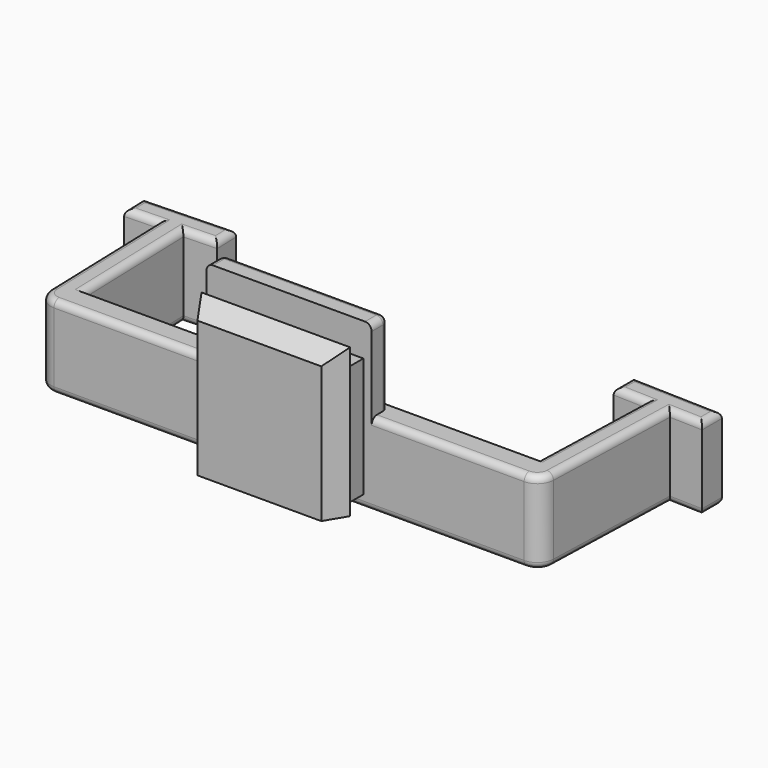
from build123d import *

# Parameters (mm, degrees)
F1_DEPTH      = 10
F3_DEPTH      = 10
F4_DEPTH      = 9
F5_DEPTH      = 9
F6_SIZE2      = 2.49999
F6_SIZE       = 1.49999
F7_R          = 0.8
F8_R          = 0.8
F9_R          = 0.8
F10_T1_DEPTH  = 10
F10_T4_ANGLE  = 88.2100893918
F10_T6_ANGLE  = 88.2100893918
F10_T8_ANGLE  = 88.2100893918
F10_T10_ANGLE = 88.2100893918


# Not quite as in the source:
# - a fillet or chamfer that OpenCascade refuses, or shapes differently, is made with other operations: its cross-section is extruded or revolved along the edge and cut away or added
# - a fillet or chamfer is up to 0.001 mm smaller than in the source, because OpenCascade refuses the exact size


with BuildPart() as f1:
    # F0 (on Top) → F1 (new body)
    with BuildSketch(Plane.XY):
        Polygon((27.5, 0), (-27.5, 0), (-28, 16), (-30.9985362283, 15.9062957429), (-30.4077144863, -3), (30.4077144863, -3), (30.9985362283, 15.9062957429), (28, 16), align=None)
        Polygon((-30.9985362283, 15.9062957429), (-28, 16), (-24.0019516957, 16.1249390095), (-24.0956559528, 19.1234752378), (-35.0902887897, 18.7798929616), (-34.9965845326, 15.7813567334), align=None)
        Polygon((24.0019516957, 16.1249390095), (28, 16), (30.9985362283, 15.9062957429), (34.9965845326, 15.7813567334), (34.9965845326, 18.7813567334), (24.0019516957, 19.1249390095), align=None)
    extrude(amount=F1_DEPTH)

    # F2 (on Right) → F3 (join, symmetric)
    with BuildSketch(Plane.YZ):
        Polygon((-3, 16), (-3, 10), (-0.5, 10), (-0.5, 20), (-3, 20), align=None)
    extrude(amount=F3_DEPTH, both=True)

    # F2 (on Right) → F4 (join, symmetric)
    with BuildSketch(Plane.YZ):
        Polygon((-3, 1.5), (-3, 10), (-3, 16), (-5, 16), (-5, 1.5), align=None)
    extrude(amount=F4_DEPTH, both=True)

    # F2 (on Right) → F5 (join, symmetric)
    with BuildSketch(Plane.YZ):
        Polygon((-5, 0), (-5, 1.5), (-5, 16), (-5, 18), (-7.5, 18), (-7.5, 0), align=None)
    extrude(amount=F5_DEPTH, both=True)

    # F6 (size 1.5 and 2.5 in the source; OpenCascade refuses exactly that, so slightly less here)
    f6_edges = [f1.edges().sort_by_distance(p)[0] for p in [
        (0, -7.5, 18),
        (-9, -7.5, 9),
        (9, -7.5, 9),
    ]]
    f6_side = f1.faces().sort_by_distance((0, -7.5, 9))[0]
    chamfer(f6_edges, length=F6_SIZE, length2=F6_SIZE2, reference=f6_side)

    # F7
    f7_edges = [f1.edges().sort_by_distance(p)[0] for p in [
        (27.75, 8, 0),
        (0, 0, 0),
        (-27.75, 8, 0),
        (-26.000976, 16.06247, 0),
        (-24.048804, 17.624207, 0),
        (-29.592972, 18.951684, 0),
        (-35.043437, 17.280625, 0),
        (-32.99756, 15.843826, 0),
        (-30.703125, 6.453148, 0),
        (0, -3, 0),
        (30.703125, 6.453148, 0),
        (32.99756, 15.843826, 0),
        (34.996585, 17.281357, 0),
        (29.499268, 18.953148, 0),
        (24.001952, 17.624939, 0),
        (26.000976, 16.06247, 0),
    ]]
    fillet(f7_edges, radius=F7_R)

    # F8
    f8_edges = [f1.edges().sort_by_distance(p)[0] for p in [
        (-29.592972, 18.951684, 10),
        (-35.043437, 17.280625, 10),
        (-32.99756, 15.843826, 10),
        (-26.000976, 16.06247, 10),
        (-24.048804, 17.624207, 10),
        (-27.75, 8, 10),
        (-30.703125, 6.453148, 10),
        (-20.203857, -3, 10),
        (20.203857, -3, 10),
        (30.703125, 6.453148, 10),
        (32.99756, 15.843826, 10),
        (34.996585, 17.281357, 10),
        (29.499268, 18.953148, 10),
        (24.001952, 17.624939, 10),
        (26.000976, 16.06247, 10),
        (27.75, 8, 10),
    ]]
    fillet(f8_edges, radius=F8_R)

    # F9
    f9_edges = [f1.edges().sort_by_distance(p)[0] for p in [
        (0, -0.5, 20),
        (-10, -0.5, 15),
        (10, -0.5, 15),
        (10, -1.75, 20),
        (-10, -1.75, 20),
    ]]
    fillet(f9_edges, radius=F9_R)

    # F10: fillet of radius 2 on 2 edges, made by hand

    # F10_s2 → F10_t1 (cut)
    with BuildSketch(Plane.XY):
        with BuildLine():
            ThreePointArc((-28.4692381621, -3), (-29.861190207, -2.4361300445), (-30.4682623143, -1.0624695048))
            Line((-30.4682623143, -1.0624695048), (-30.4077144863, -3))
            Line((-30.4077144863, -3), (-28.4692381621, -3))
        make_face()
        with BuildLine():
            ThreePointArc((28.4692381621, -3), (29.861190207, -2.4361300445), (30.4682623143, -1.0624695048))
            Line((30.4682623143, -1.0624695048), (30.4077144863, -3))
            Line((30.4077144863, -3), (28.4692381621, -3))
        make_face()
    extrude(amount=F10_T1_DEPTH, mode=Mode.SUBTRACT)

    # F10_s3 → F10_t4 (revolve, cut)
    with BuildSketch(Plane(origin=(-0.0034446457, -0.1102286623, 0), x_dir=(0, 0, 1), z_dir=(0.0312347524, 0.9995120761, 0))):
        with BuildLine():
            ThreePointArc((0, 29.6865820924), (0.2343145751, 30.2522675173), (0.8, 30.4865820924))
            Line((0.8, 30.4865820924), (0, 30.4865820924))
            Line((0, 30.4865820924), (0, 29.6865820924))
        make_face()
    revolve(axis=Axis((28.4692381621, -1, 0), (0, 0, -1)), revolution_arc=F10_T4_ANGLE, mode=Mode.SUBTRACT)

    # F10_s5 → F10_t6 (revolve, cut)
    with BuildSketch(Plane.YZ.offset(28.4692381621)):
        with BuildLine():
            ThreePointArc((-2.2, 10), (-2.7656854249, 9.7656854249), (-3, 9.2))
            Line((-3, 9.2), (-3, 10))
            Line((-3, 10), (-2.2, 10))
        make_face()
    revolve(axis=Axis((28.4692381621, -1, 10), (0, 0, 1)), revolution_arc=F10_T6_ANGLE, mode=Mode.SUBTRACT)

    # F10_s7 → F10_t8 (revolve, cut)
    with BuildSketch(Plane.YZ.offset(-28.4692381621)):
        with BuildLine():
            ThreePointArc((-2.2, 0), (-2.7656854249, 0.2343145751), (-3, 0.8))
            Line((-3, 0.8), (-3, 0))
            Line((-3, 0), (-2.2, 0))
        make_face()
    revolve(axis=Axis((-28.4692381621, -1, 0), (0, 0, -1)), revolution_arc=F10_T8_ANGLE, mode=Mode.SUBTRACT)

    # F10_s9 → F10_t10 (revolve, cut)
    with BuildSketch(Plane(origin=(0.0034446457, -0.1102286623, 0), x_dir=(0, 0, 1), z_dir=(-0.0312347524, 0.9995120761, 0))):
        with BuildLine():
            ThreePointArc((10, -29.6865820924), (9.7656854249, -30.2522675173), (9.2, -30.4865820924))
            Line((9.2, -30.4865820924), (10, -30.4865820924))
            Line((10, -30.4865820924), (10, -29.6865820924))
        make_face()
    revolve(axis=Axis((-28.4692381621, -1, 10), (0, 0, 1)), revolution_arc=F10_T10_ANGLE, mode=Mode.SUBTRACT)


solid = f1.part
